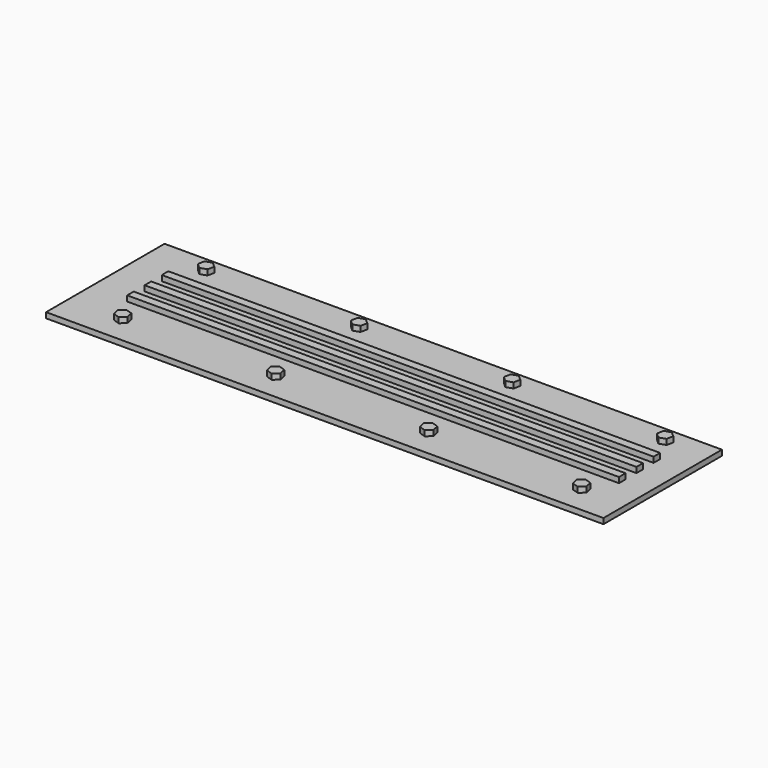
from build123d import *

# Parameters (mm, degrees)
F0_W     = 102
F0_H     = 27.1
F1_DEPTH = 1
F2_W     = 90
F2_H     = 1.5
F3_DEPTH = 1


# Not quite as in the source:
# - a feature names something its author has since deleted; it is built from what else it names


with BuildPart() as f1:
    # F0 (on Top) → F1 (new body)
    with BuildSketch(Plane.XY):
        with Locations((-1, -1)):
            Rectangle(F0_W, F0_H)
    extrude(amount=F1_DEPTH)

    # F2 (on face) → F3 (join)
    with BuildSketch(Plane.XY.offset(1)):
        Polygon((-42.2541592645, 8.3261114968), (-41.0671610971, 8.7179473687), (-40.8130018326, 9.9418358719), (-41.7458407355, 10.7738885032), (-42.9328389029, 10.3820526313), (-43.1869981674, 9.1581641281), align=None)
        Polygon((-13.0671610971, 8.7179473687), (-12.8130018326, 9.9418358719), (-13.7458407355, 10.7738885032), (-14.9328389029, 10.3820526313), (-15.1869981674, 9.1581641281), (-14.2541592645, 8.3261114968), align=None)
        Polygon((14.9328389029, 8.7179473687), (15.1869981674, 9.9418358719), (14.2541592645, 10.7738885032), (13.0671610971, 10.3820526313), (12.8130018326, 9.1581641281), (13.7458407355, 8.3261114968), align=None)
        Polygon((42.9328389029, 8.7179473687), (43.1869981674, 9.9418358719), (42.2541592645, 10.7738885032), (41.0671610971, 10.3820526313), (40.8130018326, 9.1581641281), (41.7458407355, 8.3261114968), align=None)
        Polygon((-43.1869981674, -9.1581641281), (-42.9328389029, -10.3820526313), (-41.7458407355, -10.7738885032), (-40.8130018326, -9.9418358719), (-41.0671610971, -8.7179473687), (-42.2541592645, -8.3261114968), align=None)
        Polygon((-14.2541592645, -8.3261114968), (-15.1869981674, -9.1581641281), (-14.9328389029, -10.3820526313), (-13.7458407355, -10.7738885032), (-12.8130018326, -9.9418358719), (-13.0671610971, -8.7179473687), align=None)
        Polygon((13.7458407355, -8.3261114968), (12.8130018326, -9.1581641281), (13.0671610971, -10.3820526313), (14.2541592645, -10.7738885032), (15.1869981674, -9.9418358719), (14.9328389029, -8.7179473687), align=None)
        Polygon((42.9328389029, -8.7179473687), (41.7458407355, -8.3261114968), (40.8130018326, -9.1581641281), (41.0671610971, -10.3820526313), (42.2541592645, -10.7738885032), (43.1869981674, -9.9418358719), align=None)
        with Locations((-0.065032054, 3.9994713191)):
            Rectangle(F2_W, F2_H)
        Rectangle(F2_W, F2_H)
        with Locations((0, -4)):
            Rectangle(F2_W, F2_H)
    extrude(amount=F3_DEPTH)


solid = f1.part
